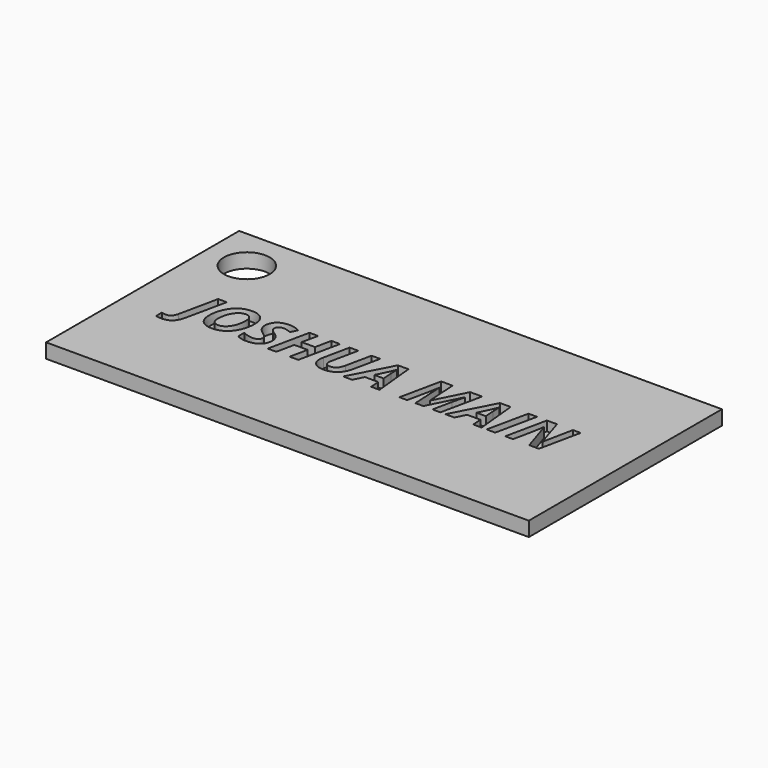
from build123d import *

# Parameters (mm, degrees)
F0_W         = 100
F0_H         = 50
F0_R         = 4.735611113
F1_DEPTH     = 3
F2_TEXT_SIZE = 11.9738072965
F3_DEPTH     = 2


# Not quite as in the source:
# - Text() gives the source's letters only with a copy of the font that has no kerning and outlines rounded to 1/6400 em; it was checked with that copy


with BuildPart() as f1:
    # F0 (on Top) → F1 (new body)
    with BuildSketch(Plane.XY):
        Rectangle(F0_W, F0_H)
        with Locations((-41.4046421647, 16.2371136248)):
            Circle(F0_R, mode=Mode.SUBTRACT)
    extrude(amount=F1_DEPTH)

    # F2 (on face) → F3 (cut)
    with BuildSketch(Plane.XY.offset(3)):
        with Locations((-40, -4.3105706268)):
            Text('JOSHUA MAIN', F2_TEXT_SIZE, font='Open Sans', font_style=FontStyle.BOLDITALIC, text_align=(TextAlign.LEFT, TextAlign.BOTTOM))
    extrude(amount=-F3_DEPTH, mode=Mode.SUBTRACT)


solid = f1.part
